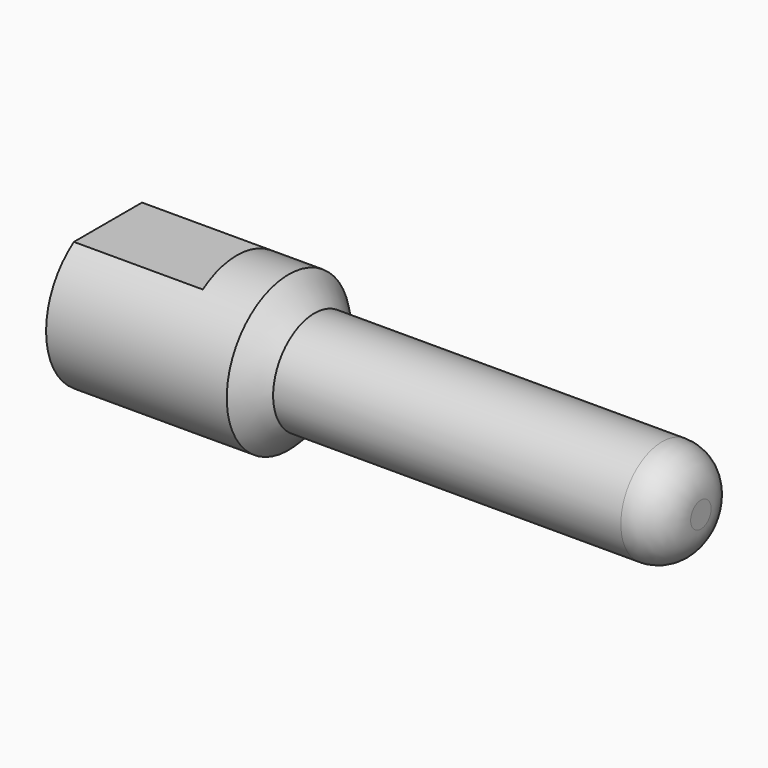
from build123d import *

# Parameters (mm, degrees)
F0_W        = 15.4432
F0_H        = 9.525
F3_DEPTH    = 15.875
F4_R        = 4.7752
F5_S5_R     = 6.35
F5_T6_DEPTH = 15
F7_D        = 8.4328
F7_DEPTH    = 19.685
F7_TIP      = 2.5334687141


# Not quite as in the source:
# - a fillet or chamfer that OpenCascade refuses, or shapes differently, is made with other operations: its cross-section is extruded or revolved along the edge and cut away or added


with BuildPart() as f1:
    # F0 (on Top) → F1 (revolve)
    with BuildSketch(Plane.XY):
        with Locations((-16.8899756006, 4.7625)):
            Rectangle(F0_W, F0_H)
        Polygon((-9.1683756006, 9.525), (-9.1683756006, 0), (48.4134243994, 0), (48.4134243994, 6.35), (0.8138243994, 6.35), (0.8138243994, 9.525), align=None)
    revolve(axis=Axis((11.9009243994, 0, 0), (1, 0, 0)))

    # F2 (on face) → F3 (cut)
    with BuildSketch(Plane(origin=(-24.6115756006, 0, 0), x_dir=(0, -1, 0), z_dir=(-1, 0, 0))):
        with BuildLine():
            ThreePointArc((5.2459455735, 7.9502), (0, 9.525), (-5.2459455735, 7.9502))
            Line((-5.2459455735, 7.9502), (5.2459455735, 7.9502))
        make_face()
        with BuildLine():
            Line((5.2651418547, -7.9375), (-5.2651418547, -7.9375))
            ThreePointArc((-5.2651418547, -7.9375), (0, -9.525), (5.2651418547, -7.9375))
        make_face()
    extrude(amount=-F3_DEPTH, mode=Mode.SUBTRACT)

    # F4
    f4_edges = [f1.edges().sort_by_distance(p)[0] for p in [
        (48.413424, -6.35, 0),
    ]]
    fillet(f4_edges, radius=F4_R)

    # F5: chamfer of 3.175 on 1 edges, made by hand


with BuildPart() as f5_tool2:
    # F5_s3 → F5_t4 (revolve)
    with BuildSketch(Plane.XY):
        Polygon((0.8138243994, 6.35), (-2.3611756006, 9.525), (0.8138243994, 9.525), align=None)
    revolve(axis=Axis((0.8138243994, 0, 0), (1, 0, 0)))

    # F5_s5 → F5_t6 (cut, symmetric)
    with BuildSketch(Plane.YZ.offset(-0.8)):
        Circle(F5_S5_R)
    extrude(amount=F5_T6_DEPTH, both=True, mode=Mode.SUBTRACT)


with BuildPart() as f1_1:
    add(f1.part)

    # F5_t1: cut F5_tool2
    add(f5_tool2.part, mode=Mode.SUBTRACT)

    # F7
    with Locations(Plane(origin=(-24.6115756006, 0, 0), x_dir=(0, -1, 0), z_dir=(-1, 0, 0))):
        with Locations((0, 0)):
            Hole(F7_D / 2, depth=F7_DEPTH)
            with Locations((0, 0, -(F7_DEPTH + F7_TIP / 2))):  # 118° drill point
                Cone(0, F7_D / 2, F7_TIP, mode=Mode.SUBTRACT)


solid = f1_1.part
